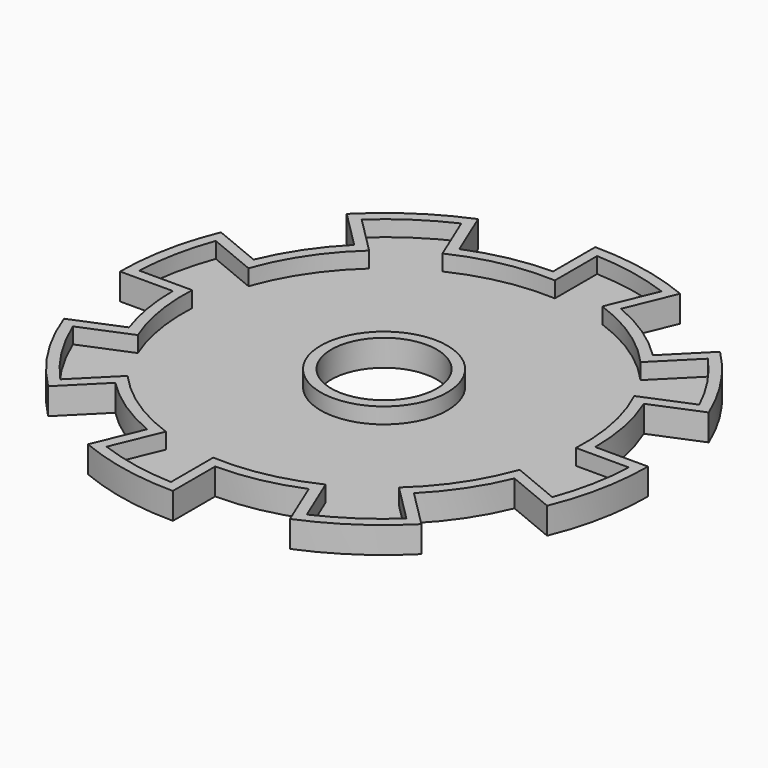
from build123d import *

# Parameters (mm, degrees)
F0_R     = 12.7
F1_DEPTH = 6.35
F2_T     = -2.54


with BuildPart() as f1:
    # F0 (on Top) → F1 (new body)
    with BuildSketch(Plane.XY):
        with BuildLine():
            Line((-46.9330802516, 19.4403183641), (-58.6663503145, 24.3003979552))
            ThreePointArc((-58.6663503145, 24.3003979552), (-62.2798653056, 12.388235448), (-63.5, 0))
            Line((-63.5, 0), (-50.8, 0))
            ThreePointArc((-50.8, 0), (-50.0884898607, -8.4724957052), (-47.9738904144, -16.7076580798))
            Line((-47.9738904144, -16.7076580798), (-59.7227298995, -21.5741867367))
            ThreePointArc((-59.7227298995, -21.5741867367), (-53.5964944807, -34.0538658507), (-44.9012806053, -44.9012806053))
            Line((-44.9012806053, -44.9012806053), (-35.9210244843, -35.9210244843))
            ThreePointArc((-35.9210244843, -35.9210244843), (-28.2229678374, -42.238656305), (-19.4403183641, -46.9330802516))
            Line((-19.4403183641, -46.9330802516), (-24.3003979552, -58.6663503145))
            ThreePointArc((-24.3003979552, -58.6663503145), (-12.388235448, -62.2798653056), (0, -63.5))
            Line((0, -63.5), (0, -50.8))
            ThreePointArc((0, -50.8), (9.9105883584, -49.8238922445), (19.4403183641, -46.9330802516))
            Line((19.4403183641, -46.9330802516), (24.3003979552, -58.6663503145))
            ThreePointArc((24.3003979552, -58.6663503145), (35.2787097967, -52.7983203812), (44.9012806053, -44.9012806053))
            Line((44.9012806053, -44.9012806053), (35.9210244843, -35.9210244843))
            ThreePointArc((35.9210244843, -35.9210244843), (42.238656305, -28.2229678374), (46.9330802516, -19.4403183641))
            Line((46.9330802516, -19.4403183641), (58.6663503145, -24.3003979552))
            ThreePointArc((58.6663503145, -24.3003979552), (62.2798653056, -12.388235448), (63.5, 0))
            Line((63.5, 0), (50.8, 0))
            ThreePointArc((50.8, 0), (49.8238922445, 9.9105883584), (46.9330802516, 19.4403183641))
            Line((46.9330802516, 19.4403183641), (58.6663503145, 24.3003979552))
            ThreePointArc((58.6663503145, 24.3003979552), (52.7983203812, 35.2787097967), (44.9012806053, 44.9012806053))
            Line((44.9012806053, 44.9012806053), (35.9210244843, 35.9210244843))
            ThreePointArc((35.9210244843, 35.9210244843), (28.2229678374, 42.238656305), (19.4403183641, 46.9330802516))
            Line((19.4403183641, 46.9330802516), (24.3003979552, 58.6663503145))
            ThreePointArc((24.3003979552, 58.6663503145), (12.388235448, 62.2798653056), (0, 63.5))
            Line((0, 63.5), (0, 50.8))
            ThreePointArc((0, 50.8), (-9.9105883584, 49.8238922445), (-19.4403183641, 46.9330802516))
            Line((-19.4403183641, 46.9330802516), (-24.3003979552, 58.6663503145))
            ThreePointArc((-24.3003979552, 58.6663503145), (-35.2787097967, 52.7983203812), (-44.9012806053, 44.9012806053))
            Line((-44.9012806053, 44.9012806053), (-35.9210244843, 35.9210244843))
            ThreePointArc((-35.9210244843, 35.9210244843), (-42.238656305, 28.2229678374), (-46.9330802516, 19.4403183641))
        make_face()
        Circle(F0_R, mode=Mode.SUBTRACT)
    extrude(amount=F1_DEPTH)

    # F2
    f2_openings = [f1.faces().sort_by_distance(p)[0] for p in [
        (-34.280877, 51.304958, 6.35),
    ]]
    offset(amount=F2_T, openings=f2_openings, kind=Kind.INTERSECTION)


solid = f1.part
